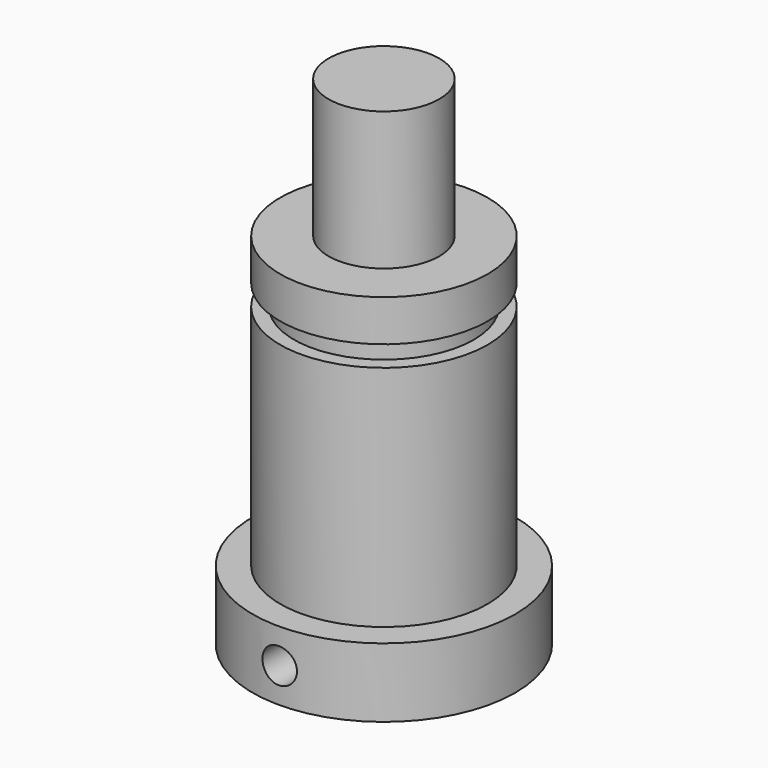
from build123d import *

# Parameters (mm, degrees)
F0_R      = 7.5
F1_DEPTH  = 21
F2_R      = 9.5
F3_DEPTH  = 5
F5_D      = 6.35
F5_DEPTH  = 15
F5_TIP    = 1.9077324654
F7_D      = 2.5
F7_DEPTH  = 9.501
F8_R      = 7.5
F9_DEPTH  = 5
F10_R     = 4
F11_DEPTH = 10
F13_R     = 7.5
F13_R_2   = 6.5
F14_DEPTH = 1.5


with BuildPart() as f1:
    # F0 (on Top) → F1 (new body)
    with BuildSketch(Plane.XY):
        Circle(F0_R)
    extrude(amount=F1_DEPTH)

    # F2 (on Top) → F3 (join)
    with BuildSketch(Plane.XY):
        Circle(F2_R)
    extrude(amount=F3_DEPTH)

    # F5
    with Locations(Plane(origin=(0, 0, 0), x_dir=(1, 0, 0), z_dir=(0, 0, -1))):
        with Locations((0, 0)):
            Hole(F5_D / 2, depth=F5_DEPTH)
            with Locations((0, 0, -(F5_DEPTH + F5_TIP / 2))):  # 118° drill point
                Cone(0, F5_D / 2, F5_TIP, mode=Mode.SUBTRACT)

    # F7 (through all, one way)
    with BuildSketch(Plane(origin=(0, 0, 0), x_dir=(1, 0, 0), z_dir=(0, 1, 0))):
        with Locations((0, -2.5)):
            Circle(F7_D / 2)
    extrude(amount=-F7_DEPTH, mode=Mode.SUBTRACT)

    # F8 (on face) → F9 (join)
    with BuildSketch(Plane.XY.offset(21)):
        Circle(F8_R)
    extrude(amount=F9_DEPTH)

    # F10 (on face) → F11 (join)
    with BuildSketch(Plane.XY.offset(26)):
        Circle(F10_R)
    extrude(amount=F11_DEPTH)

    # F13 (on offset) → F14 (cut)
    with BuildSketch(Plane.XY.offset(21.5)):
        Circle(F13_R)
        Circle(F13_R_2, mode=Mode.SUBTRACT)
    extrude(amount=F14_DEPTH, mode=Mode.SUBTRACT)


solid = f1.part
